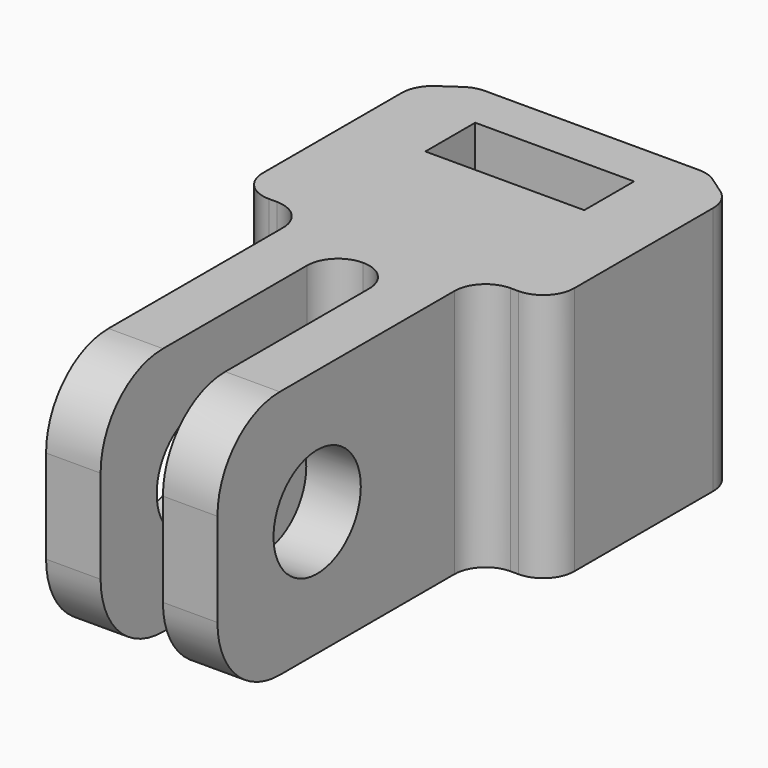
from build123d import *

# Parameters (mm, degrees)
F1_DEPTH  = 16
F2_R      = 2.5
F3_DEPTH  = 12
F4_R      = 3.5
F5_DEPTH  = 11
F6_R      = 1.99999
F7_W      = 10.2
F7_H      = 4
F8_DEPTH  = 12.3
F9_R      = 5
F10_W     = 9.5
F10_H     = 9.5
F10_R     = 2.05
F11_DEPTH = 3.2
F12_R     = 2


# Not quite as in the source:
# - a fillet or chamfer is up to 0.001 mm smaller than in the source, because OpenCascade refuses the exact size


with BuildPart() as f1:
    # F0 (on Top) → F1 (new body)
    with BuildSketch(Plane.XY):
        Polygon((-5.5, -4.9891225062), (-5.5, -26), (-2, -26), (-2, -7.4497503303), (2, -7.4497503303), (2, -26), (5.5, -26), (5.5, -4.9891225062), (10, -4.9891225062), (10, 9.1980283093), (7.5, 10.9290892892), (-7.5, 10.9290892892), (-10, 9.1980283093), (-10, -4.9891225062), align=None)
    extrude(amount=F1_DEPTH)

    # F2 (on face) → F3 (cut)
    with BuildSketch(Plane(origin=(0, 10.9290892892, 0), x_dir=(-1, 0, 0), z_dir=(0, 1, 0))):
        with Locations((0, 9)):
            Circle(F2_R)
    extrude(amount=-F3_DEPTH, mode=Mode.SUBTRACT)

    # F4 (on face) → F5 (cut, through all)
    with BuildSketch(Plane.YZ.offset(5.5)):
        with Locations((-18, 8)):
            Circle(F4_R)
    extrude(amount=-F5_DEPTH, mode=Mode.SUBTRACT)

    # F6 (radius 2 in the source; OpenCascade refuses exactly that, so slightly less here)
    f6_edges = [f1.edges().sort_by_distance(p)[0] for p in [
        (-5.5, -4.989123, 8),
        (2, -7.44975, 8),
        (-2, -7.44975, 8),
        (5.5, -4.989123, 8),
    ]]
    fillet(f6_edges, radius=F6_R)

    # F7 (on face) → F8 (cut)
    with BuildSketch(Plane.XY.offset(16)):
        with Locations((0, 5.9290892892)):
            Rectangle(F7_W, F7_H)
    extrude(amount=-F8_DEPTH, mode=Mode.SUBTRACT)

    # F9
    f9_edges = [f1.edges().sort_by_distance(p)[0] for p in [
        (3.75, -26, 16),
        (3.75, -26, 0),
        (-3.75, -26, 16),
        (-3.75, -26, 0),
    ]]
    fillet(f9_edges, radius=F9_R)

    # F12
    f12_edges = [f1.edges().sort_by_distance(p)[0] for p in [
        (-10, -4.989123, 8),
        (10, -4.989123, 8),
        (-10, 9.198028, 8),
        (-7.5, 10.929089, 8),
        (7.5, 10.929089, 8),
        (10, 9.198028, 8),
    ]]
    fillet(f12_edges, radius=F12_R)


with BuildPart() as f11:
    # F10 (on face) → F11 (new body)
    with BuildSketch(Plane(origin=(0, 3.9290892892, 0), x_dir=(-1, 0, 0), z_dir=(0, 1, 0))):
        with Locations((0, 9)):
            Rectangle(F10_W, F10_H)
        with Locations((0, 9)):
            Circle(F10_R, mode=Mode.SUBTRACT)
    extrude(amount=F11_DEPTH)


solid = Compound([f1.part, f11.part])
